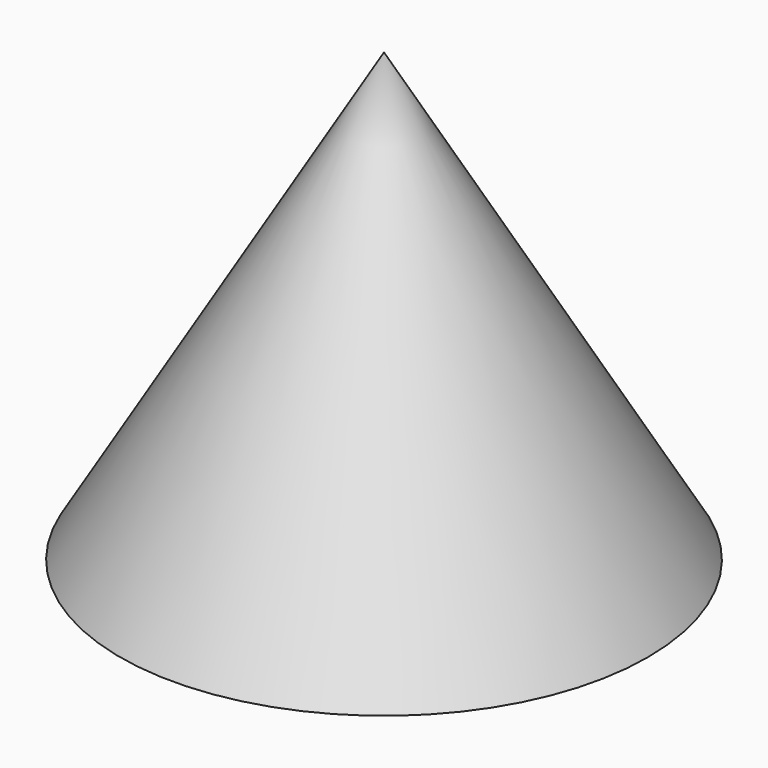
from build123d import *


# Not quite as in the source:
# - the program builds the solid bodies; features that only make, move or delete a surface that nothing else refers to are left out


with BuildPart() as f1:
    # F0 (on Front) → F1 (revolve)
    with BuildSketch(Plane.XZ):
        Polygon((-13.9187909663, -2.4887903128), (-34.9352434278, 33.0916941166), (-34.9352434278, -2.4887903128), align=None)
    revolve(axis=Axis((-34.9352434278, 0, 15.3014519019), (0, 0, -1)))


solid = f1.part
